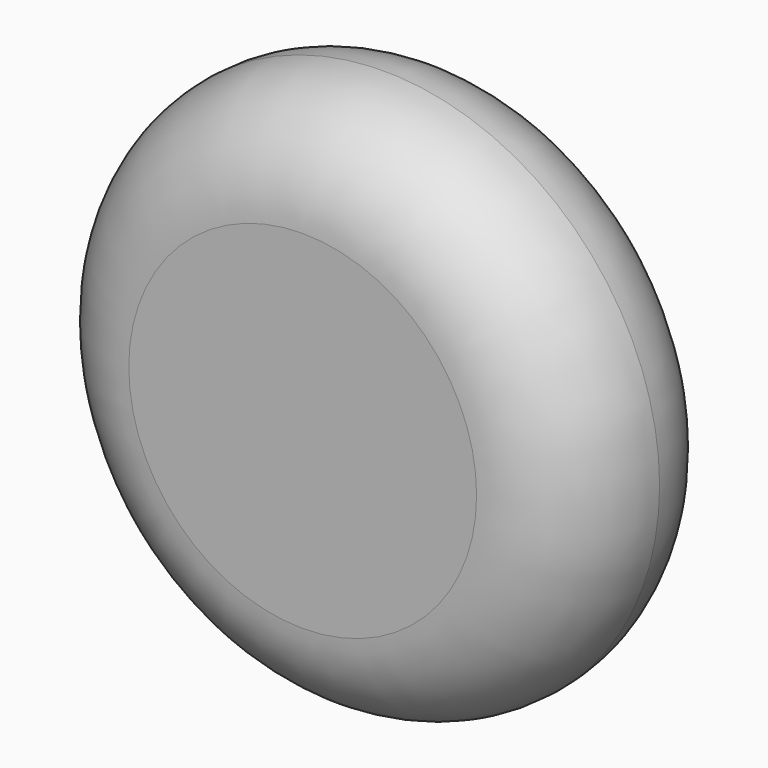
from build123d import *

# Parameters (mm, degrees)
F0_R     = 34.4282754843
F1_DEPTH = 25.4
F2_R     = 12.69999


# Not quite as in the source:
# - a fillet or chamfer is up to 0.001 mm smaller than in the source, because OpenCascade refuses the exact size


with BuildPart() as f1:
    # F0 (on Front) → F1 (new body)
    with BuildSketch(Plane.XZ):
        Circle(F0_R)
    extrude(amount=F1_DEPTH)

    # F2 (radius 12.7 in the source; OpenCascade refuses exactly that, so slightly less here)
    f2_edges = [f1.edges().sort_by_distance(p)[0] for p in [
        (34.428275, -12.7, 0),
        (-34.428275, 0, 0),
        (-34.428275, -25.4, 0),
    ]]
    fillet(f2_edges, radius=F2_R)


solid = f1.part
